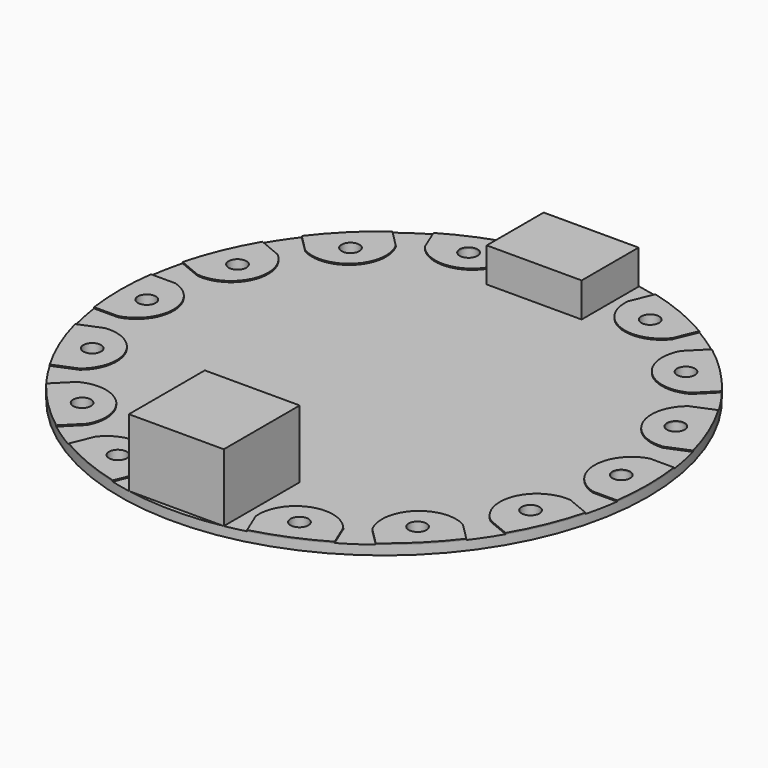
from build123d import *

# Parameters (mm, degrees)
F0_R             = 22.25
F1_DEPTH         = 0.8
F2_W             = 8
F2_H             = 8
F3_DEPTH         = 5.7
F4_W             = 8
F4_H             = 6
F5_DEPTH         = 2.9
F6_R             = 0.75
F7_DEPTH         = 0.8
F7_COPIES_COUNT  = 4
F7_COPIES_ANGLE  = 67.5
F7_COPIES1_COUNT = 4
F7_COPIES1_ANGLE = 337.5
F7_COPIES2_COUNT = 3
F7_COPIES2_ANGLE = 315
F7_COPIES3_COUNT = 3
F7_COPIES3_ANGLE = 225
F8_DEPTH         = 0.1
F8_COPIES_COUNT  = 4
F8_COPIES_ANGLE  = 67.5
F8_COPIES1_COUNT = 4
F8_COPIES1_ANGLE = 337.5
F8_COPIES2_COUNT = 3
F8_COPIES2_ANGLE = 315
F8_COPIES3_COUNT = 3
F8_COPIES3_ANGLE = 225


# Not quite as in the source:
# - after a boolean that leaves OpenCascade's solid faulty, fix() repairs it
# - a feature of the source that left no trace in its solid (it failed there, or was rolled back) is left out
# - a pattern or mirror of a feature is missing from the dataset's text; its kind, count and spacing are read off the source's solid


with BuildPart() as f1:
    # F0 (on Top) → F1 (new body)
    with BuildSketch(Plane.XY):
        Circle(F0_R)
    extrude(amount=F1_DEPTH)

    # F2 (on face) → F3 (join)
    with BuildSketch(Plane.XY.offset(0.8)):
        with Locations((0, -17.8874964306)):
            Rectangle(F2_W, F2_H)
    extrude(amount=F3_DEPTH)

    # F4 (on face) → F5 (join)
    with BuildSketch(Plane.XY.offset(0.8)):
        with Locations((0, 18.82292144)):
            Rectangle(F4_W, F4_H)
    extrude(amount=F5_DEPTH)

    # F6 (on face) → F7 (cut, through all)
    with BuildSketch(Plane.XY.offset(0.8)):
        with Locations((-20, 0)):
            Circle(F6_R)
    f7 = extrude(amount=-F7_DEPTH, mode=Mode.SUBTRACT)

    # F7_copies: F7 ×4 about axis
    f7_copies_axis = Axis((0, 0, 0), (0, 0, 1))
    for i in range(1, F7_COPIES_COUNT):
        add(f7.rotate(f7_copies_axis, i * F7_COPIES_ANGLE / (F7_COPIES_COUNT - 1)), mode=Mode.SUBTRACT)

    # F7_copies1: F7 ×4 about axis
    f7_copies1_axis = Axis((0, 0, 0), (0, 0, 1))
    for i in range(1, F7_COPIES1_COUNT):
        add(f7.rotate(f7_copies1_axis, i * F7_COPIES1_ANGLE / (F7_COPIES1_COUNT - 1)), mode=Mode.SUBTRACT)

    # F7_copies2: F7 ×3 about axis
    f7_copies2_axis = Axis((0, 0, 0), (0, 0, 1))
    for i in range(1, F7_COPIES2_COUNT):
        add(f7.rotate(f7_copies2_axis, i * F7_COPIES2_ANGLE / (F7_COPIES2_COUNT - 1)), mode=Mode.SUBTRACT)

    # F7_copies3: F7 ×3 about axis
    f7_copies3_axis = Axis((0, 0, 0), (0, 0, -1))
    for i in range(1, F7_COPIES3_COUNT):
        add(f7.rotate(f7_copies3_axis, i * F7_COPIES3_ANGLE / (F7_COPIES3_COUNT - 1)), mode=Mode.SUBTRACT)

    # F7_copies4: F7 across plane
    add(f7.mirror(Plane(origin=(0, 0, 0), x_dir=(-0.195090322, 0.9807852804, 0), z_dir=(0.9807852804, 0.195090322, 0))), mode=Mode.SUBTRACT)

    # F7_copies5: F7 across plane
    add(f7.mirror(Plane(origin=(0, 0, 0), x_dir=(0.8314696123, -0.555570233, 0), z_dir=(0.555570233, 0.8314696123, 0))), mode=Mode.SUBTRACT)

    # F7_copies6: F7 across plane
    add(f7.mirror(Plane(origin=(0, 0, 0), x_dir=(0, 0, 1), z_dir=(1, 0, 0))), mode=Mode.SUBTRACT)

    # F6 (on face) → F8 (join)
    with BuildSketch(Plane.XY.offset(0.8)):
        with BuildLine():
            Line((-22.0468251683, -3), (-20, -3))
            ThreePointArc((-20, -3), (-17.75, 0), (-20, 3))
            Line((-20, 3), (-22.0468251683, 3))
            ThreePointArc((-22.0468251683, 3), (-22.25, 0), (-22.0468251683, -3))
        make_face()
        with Locations((-20, 0)):
            Circle(F6_R, mode=Mode.SUBTRACT)
    f8 = extrude(amount=F8_DEPTH)

    # F8_copies: F8 ×4 about axis
    f8_copies_axis = Axis((0, 0, 0), (0, 0, 1))
    for i in range(1, F8_COPIES_COUNT):
        add(f8.rotate(f8_copies_axis, i * F8_COPIES_ANGLE / (F8_COPIES_COUNT - 1)))

    # F8_copies1: F8 ×4 about axis
    f8_copies1_axis = Axis((0, 0, 0), (0, 0, 1))
    for i in range(1, F8_COPIES1_COUNT):
        add(f8.rotate(f8_copies1_axis, i * F8_COPIES1_ANGLE / (F8_COPIES1_COUNT - 1)))

    # F8_copies2: F8 ×3 about axis
    f8_copies2_axis = Axis((0, 0, 0), (0, 0, 1))
    for i in range(1, F8_COPIES2_COUNT):
        add(f8.rotate(f8_copies2_axis, i * F8_COPIES2_ANGLE / (F8_COPIES2_COUNT - 1)))

    # F8_copies3: F8 ×3 about axis
    f8_copies3_axis = Axis((0, 0, 0), (0, 0, -1))
    for i in range(1, F8_COPIES3_COUNT):
        add(f8.rotate(f8_copies3_axis, i * F8_COPIES3_ANGLE / (F8_COPIES3_COUNT - 1)))

    # F8_copies4: F8 across plane
    add(f8.mirror(Plane(origin=(0, 0, 0), x_dir=(-0.195090322, 0.9807852804, 0), z_dir=(0.9807852804, 0.195090322, 0))))

    # F8_copies5: F8 across plane
    add(f8.mirror(Plane(origin=(0, 0, 0), x_dir=(0.8314696123, -0.555570233, 0), z_dir=(0.555570233, 0.8314696123, 0))))

    add(f1.part.fix(), mode=Mode.REPLACE)

    # F8_copies6: F8 across plane
    add(f8.mirror(Plane(origin=(0, 0, 0), x_dir=(0, 0, 1), z_dir=(1, 0, 0))))


solid = f1.part
